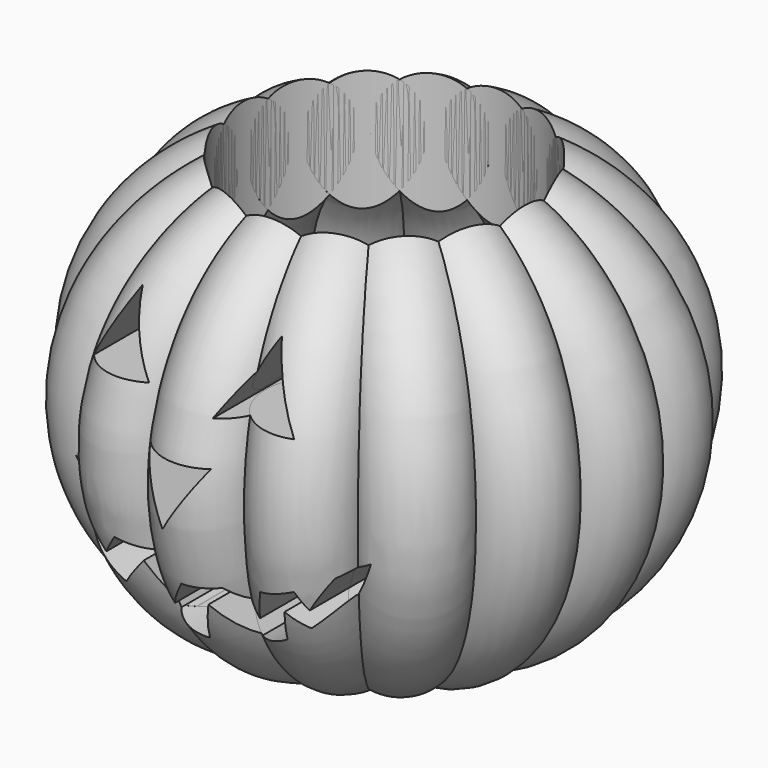
from build123d import *

# Parameters (mm, degrees)
F2_R      = 22.225
F5_COUNT  = 16
F9_DEPTH  = 127
F10_R     = 63.5
F11_DEPTH = 101.6


with BuildPart() as f3:
    # F3: sweep along a path in F0
    with BuildLine(Plane.XZ) as f3_path:
        ThreePointArc((0, 79.1287273169), (-97.8956622285, 0), (0, -79.1287273169))
    # F2 (on plane+point) → F3 (sweep)
    with BuildSketch(Plane.YZ):
        with Locations((0, 79.1287273169)):
            Circle(F2_R)
    sweep(path=f3_path.line)


with BuildPart() as f5_1:
    # F5: instance of F3
    add(f3.part.rotate(Axis((0, 0, 18.890734762), (0, 0, 1)), 1 * 360 / F5_COUNT))


with BuildPart() as f5_2:
    # F5: instance of F3
    add(f3.part.rotate(Axis((0, 0, 18.890734762), (0, 0, 1)), 2 * 360 / F5_COUNT))


with BuildPart() as f5_3:
    # F5: instance of F3
    add(f3.part.rotate(Axis((0, 0, 18.890734762), (0, 0, 1)), 3 * 360 / F5_COUNT))


with BuildPart() as f5_4:
    # F5: instance of F3
    add(f3.part.rotate(Axis((0, 0, 18.890734762), (0, 0, 1)), 4 * 360 / F5_COUNT))


with BuildPart() as f5_5:
    # F5: instance of F3
    add(f3.part.rotate(Axis((0, 0, 18.890734762), (0, 0, 1)), 5 * 360 / F5_COUNT))


with BuildPart() as f5_6:
    # F5: instance of F3
    add(f3.part.rotate(Axis((0, 0, 18.890734762), (0, 0, 1)), 6 * 360 / F5_COUNT))


with BuildPart() as f5_7:
    # F5: instance of F3
    add(f3.part.rotate(Axis((0, 0, 18.890734762), (0, 0, 1)), 7 * 360 / F5_COUNT))


with BuildPart() as f5_8:
    # F5: instance of F3
    add(f3.part.rotate(Axis((0, 0, 18.890734762), (0, 0, 1)), 8 * 360 / F5_COUNT))


with BuildPart() as f5_9:
    # F5: instance of F3
    add(f3.part.rotate(Axis((0, 0, 18.890734762), (0, 0, 1)), 9 * 360 / F5_COUNT))


with BuildPart() as f5_10:
    # F5: instance of F3
    add(f3.part.rotate(Axis((0, 0, 18.890734762), (0, 0, 1)), 10 * 360 / F5_COUNT))


with BuildPart() as f5_11:
    # F5: instance of F3
    add(f3.part.rotate(Axis((0, 0, 18.890734762), (0, 0, 1)), 11 * 360 / F5_COUNT))


with BuildPart() as f5_12:
    # F5: instance of F3
    add(f3.part.rotate(Axis((0, 0, 18.890734762), (0, 0, 1)), 12 * 360 / F5_COUNT))


with BuildPart() as f5_13:
    # F5: instance of F3
    add(f3.part.rotate(Axis((0, 0, 18.890734762), (0, 0, 1)), 13 * 360 / F5_COUNT))


with BuildPart() as f5_14:
    # F5: instance of F3
    add(f3.part.rotate(Axis((0, 0, 18.890734762), (0, 0, 1)), 14 * 360 / F5_COUNT))


with BuildPart() as f5_15:
    # F5: instance of F3
    add(f3.part.rotate(Axis((0, 0, 18.890734762), (0, 0, 1)), 15 * 360 / F5_COUNT))


with BuildPart() as f9_tool:
    # F8 (on offset) → F9 (new body)
    with BuildSketch(Plane.XZ.offset(127)):
        Polygon((-36.8289723992, 64.1175955534), (-51.9780814648, 34.8514541984), (-23.4711002558, 34.8514541984), align=None)
        Polygon((26.4032335243, 64.4347148861), (11.0899731517, 34.8514541984), (43.4565804899, 34.8514541984), align=None)
        with BuildLine():
            Line((-52.8587867229, -20.8229999341), (-66.5405392647, -13.1553560495))
            ThreePointArc((-66.5405392647, -13.1553560495), (-54.3000925565, -33.8199285917), (-35.8884493374, -49.2427846158))
            Line((-35.8884493374, -49.2427846158), (-25.3525711596, -36.1284911633))
            Line((-25.3525711596, -36.1284911633), (-17.4355855756, -56.7758259758))
            ThreePointArc((-17.4355855756, -56.7758259758), (-7.609335954, -58.5347469197), (2.3663042484, -58.9029684079))
            Line((2.3663042484, -58.9029684079), (8.5129486397, -40.2334034443))
            Line((8.5129486397, -40.2334034443), (18.7247998978, -56.4375618124))
            ThreePointArc((18.7247998978, -56.4375618124), (28.1040665009, -53.164823919), (36.9369361244, -48.6192909971))
            Line((36.9369361244, -48.6192909971), (40.0694571435, -34.3325920403))
            Line((40.0694571435, -34.3325920403), (47.2667594041, -41.0045659964))
            ThreePointArc((47.2667594041, -41.0045659964), (58.5825906839, -28.2419166415), (66.5405392647, -13.1553560495))
            ThreePointArc((66.5405392647, -13.1553560495), (61.6276289249, -16.1767911073), (56.5778006507, -18.9633646691))
            Line((56.5778006507, -18.9633646691), (48.7923957407, -32.2801358998))
            Line((48.7923957407, -32.2801358998), (45.4961947383, -24.0565059319))
            ThreePointArc((45.4961947383, -24.0565059319), (37.9357256061, -26.7999044286), (30.2113664998, -29.0407090183))
            Line((30.2113664998, -29.0407090183), (24.6760398149, -44.0817549825))
            Line((24.6760398149, -44.0817549825), (14.3908314725, -31.9797084935))
            ThreePointArc((14.3908314725, -31.9797084935), (7.2079317689, -32.6164021283), (0, -32.828879307))
            Line((0, -32.828879307), (-9.4460388646, -46.9038821757))
            Line((-9.4460388646, -46.9038821757), (-18.567500251, -31.4119690224))
            ThreePointArc((-18.567500251, -31.4119690224), (-26.68249849, -29.8842960421), (-34.6759857793, -27.8127888346))
            Line((-34.6759857793, -27.8127888346), (-41.5156595409, -37.4112762511))
            Line((-41.5156595409, -37.4112762511), (-52.8587867229, -20.8229999341))
        make_face()
        Polygon((-18.3969289064, 16.8077480048), (-5.1251077093, -11.108844541), (13.1808547303, 16.8077480048), align=None)
    extrude(amount=-F9_DEPTH)


with BuildPart() as f3_1:
    add(f3.part)

    # F9: cut by f9_tool
    add(f9_tool.part, mode=Mode.SUBTRACT)


with BuildPart() as f5_1_1:
    add(f5_1.part)

    # F9: cut by f9_tool
    add(f9_tool.part, mode=Mode.SUBTRACT)


with BuildPart() as f5_2_1:
    add(f5_2.part)

    # F9: cut by f9_tool
    add(f9_tool.part, mode=Mode.SUBTRACT)


with BuildPart() as f5_3_1:
    add(f5_3.part)

    # F9: cut by f9_tool
    add(f9_tool.part, mode=Mode.SUBTRACT)


with BuildPart() as f5_4_1:
    add(f5_4.part)

    # F9: cut by f9_tool
    add(f9_tool.part, mode=Mode.SUBTRACT)


with BuildPart() as f5_5_1:
    add(f5_5.part)

    # F9: cut by f9_tool
    add(f9_tool.part, mode=Mode.SUBTRACT)


with BuildPart() as f5_6_1:
    add(f5_6.part)

    # F9: cut by f9_tool
    add(f9_tool.part, mode=Mode.SUBTRACT)


with BuildPart() as f5_7_1:
    add(f5_7.part)

    # F9: cut by f9_tool
    add(f9_tool.part, mode=Mode.SUBTRACT)


with BuildPart() as f5_8_1:
    add(f5_8.part)

    # F9: cut by f9_tool
    add(f9_tool.part, mode=Mode.SUBTRACT)


with BuildPart() as f5_9_1:
    add(f5_9.part)

    # F9: cut by f9_tool
    add(f9_tool.part, mode=Mode.SUBTRACT)


with BuildPart() as f5_15_1:
    add(f5_15.part)

    # F9: cut by f9_tool
    add(f9_tool.part, mode=Mode.SUBTRACT)


with BuildPart() as f11_tool:
    # F10 (on offset) → F11 (new body)
    with BuildSketch(Plane.XY.offset(127)):
        Circle(F10_R)
    extrude(amount=-F11_DEPTH)


with BuildPart() as f3_2:
    add(f3_1.part)

    # F11: cut by f11_tool
    add(f11_tool.part, mode=Mode.SUBTRACT)


with BuildPart() as f5_1_2:
    add(f5_1_1.part)

    # F11: cut by f11_tool
    add(f11_tool.part, mode=Mode.SUBTRACT)


with BuildPart() as f5_2_2:
    add(f5_2_1.part)

    # F11: cut by f11_tool
    add(f11_tool.part, mode=Mode.SUBTRACT)


with BuildPart() as f5_3_2:
    add(f5_3_1.part)

    # F11: cut by f11_tool
    add(f11_tool.part, mode=Mode.SUBTRACT)


with BuildPart() as f5_4_2:
    add(f5_4_1.part)

    # F11: cut by f11_tool
    add(f11_tool.part, mode=Mode.SUBTRACT)


with BuildPart() as f5_5_2:
    add(f5_5_1.part)

    # F11: cut by f11_tool
    add(f11_tool.part, mode=Mode.SUBTRACT)


with BuildPart() as f5_6_2:
    add(f5_6_1.part)

    # F11: cut by f11_tool
    add(f11_tool.part, mode=Mode.SUBTRACT)


with BuildPart() as f5_7_2:
    add(f5_7_1.part)

    # F11: cut by f11_tool
    add(f11_tool.part, mode=Mode.SUBTRACT)


with BuildPart() as f5_8_2:
    add(f5_8_1.part)

    # F11: cut by f11_tool
    add(f11_tool.part, mode=Mode.SUBTRACT)


with BuildPart() as f5_9_2:
    add(f5_9_1.part)

    # F11: cut by f11_tool
    add(f11_tool.part, mode=Mode.SUBTRACT)


with BuildPart() as f5_10_1:
    add(f5_10.part)

    # F11: cut by f11_tool
    add(f11_tool.part, mode=Mode.SUBTRACT)


with BuildPart() as f5_11_1:
    add(f5_11.part)

    # F11: cut by f11_tool
    add(f11_tool.part, mode=Mode.SUBTRACT)


with BuildPart() as f5_12_1:
    add(f5_12.part)

    # F11: cut by f11_tool
    add(f11_tool.part, mode=Mode.SUBTRACT)


with BuildPart() as f5_13_1:
    add(f5_13.part)

    # F11: cut by f11_tool
    add(f11_tool.part, mode=Mode.SUBTRACT)


with BuildPart() as f5_14_1:
    add(f5_14.part)

    # F11: cut by f11_tool
    add(f11_tool.part, mode=Mode.SUBTRACT)


with BuildPart() as f5_15_2:
    add(f5_15_1.part)

    # F11: cut by f11_tool
    add(f11_tool.part, mode=Mode.SUBTRACT)


solid = Compound([f3_2.part, f5_1_2.part, f5_2_2.part, f5_3_2.part, f5_4_2.part, f5_5_2.part, f5_6_2.part, f5_7_2.part, f5_8_2.part, f5_9_2.part, f5_10_1.part, f5_11_1.part, f5_12_1.part, f5_13_1.part, f5_14_1.part, f5_15_2.part])
